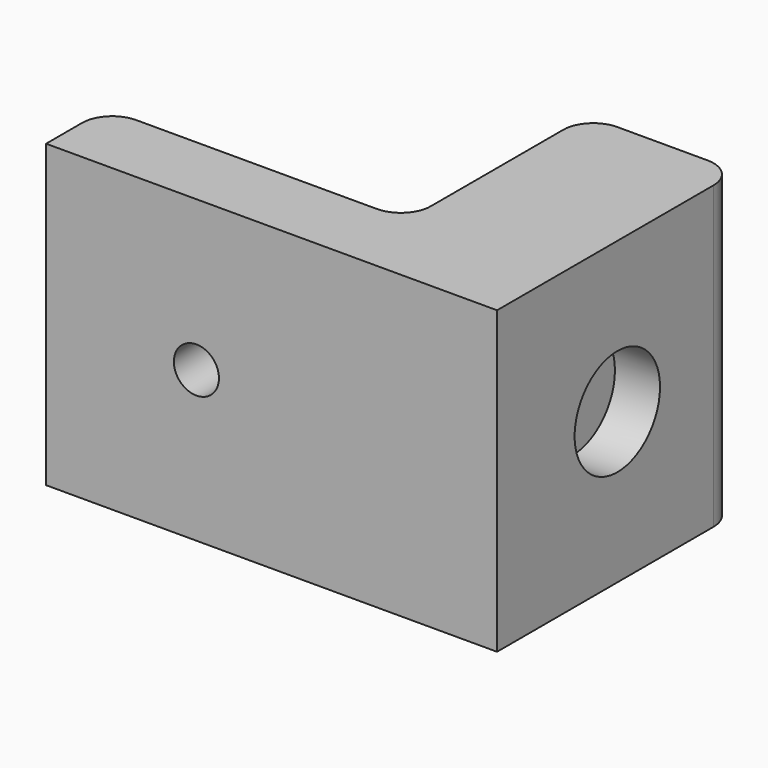
from build123d import *

# Parameters (mm, degrees)
F1_DEPTH     = 20
F2_R         = 3.55
F3_DEPTH     = 3
F4_R         = 1.5
F5_DEPTH     = 25
F6_R         = 2
F7_TEXT_SIZE = 4.2588587589
F8_DEPTH     = 0.4


# Not quite as in the source:
# - Text() gives the source's letters only with a copy of the font that has no kerning and outlines rounded to 1/6400 em; it was checked with that copy


with BuildPart() as f1:
    # F0 (on Top) → F1 (new body)
    with BuildSketch(Plane.XY):
        Polygon((20, 15), (20, 0), (0, 0), (0, -5), (30, -5), (30, 15), align=None)
    extrude(amount=F1_DEPTH)

    # F2 (on face) → F3 (cut)
    with BuildSketch(Plane.YZ.offset(30)):
        with Locations((5, 10)):
            Circle(F2_R)
    extrude(amount=-F3_DEPTH, mode=Mode.SUBTRACT)

    # F4 (on face) → F5 (cut)
    with BuildSketch(Plane(origin=(0, 0, 0), x_dir=(-1, 0, 0), z_dir=(0, 1, 0))):
        with Locations((-10, 10)):
            Circle(F4_R)
    extrude(amount=-F5_DEPTH, mode=Mode.SUBTRACT)

    # F6
    f6_edges = [f1.edges().sort_by_distance(p)[0] for p in [
        (20, 0, 10),
        (0, 0, 10),
        (30, 15, 10),
        (20, 15, 10),
    ]]
    fillet(f6_edges, radius=F6_R)


with BuildPart() as f8:
    # F7 (on face) → F8 (new body)
    with BuildSketch(Plane(origin=(0, 15, 0), x_dir=(-1, 0, 0), z_dir=(0, 1, 0))):
        with Locations(Location((-23.5, 2), (0, 0, 90))):
            Text('SIKORA', F7_TEXT_SIZE, font='Open Sans', font_style=FontStyle.BOLD, text_align=(TextAlign.LEFT, TextAlign.BOTTOM))
    extrude(amount=F8_DEPTH)


solid = Compound([f1.part, f8.part])
